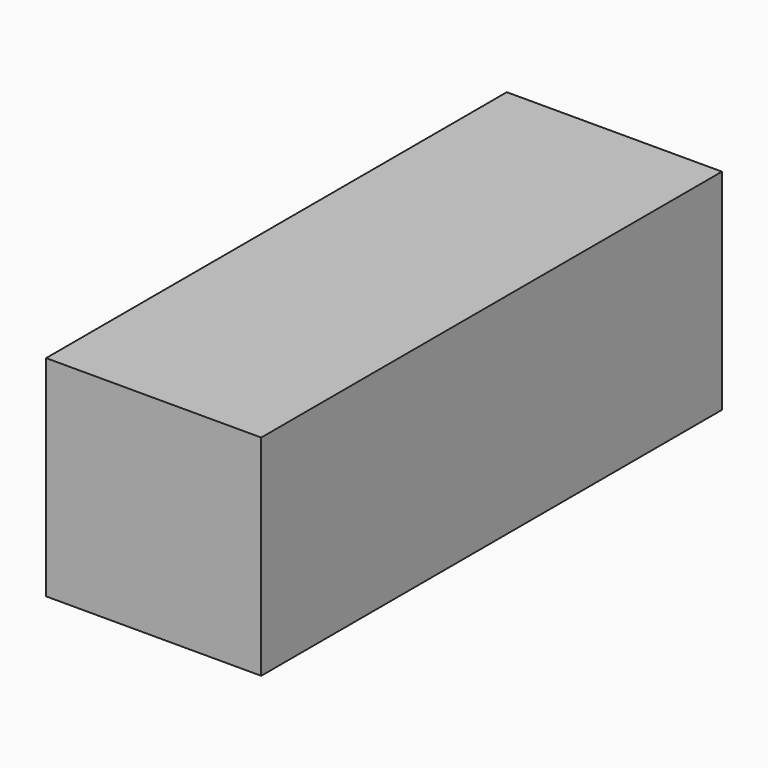
from build123d import *

# Parameters (mm, degrees)
F2_W     = 66.9259168208
F2_H     = 24.3781767786
F3_DEPTH = 25


# Not quite as in the source:
# - the program builds the solid bodies; features that only make, move or delete a surface that nothing else refers to are left out


with BuildPart() as f3:
    # F2 (on Right) → F3 (new body)
    with BuildSketch(Plane.YZ):
        with Locations((75.2753894776, 27.9002320021)):
            Rectangle(F2_W, F2_H)
    extrude(amount=F3_DEPTH)


solid = f3.part
